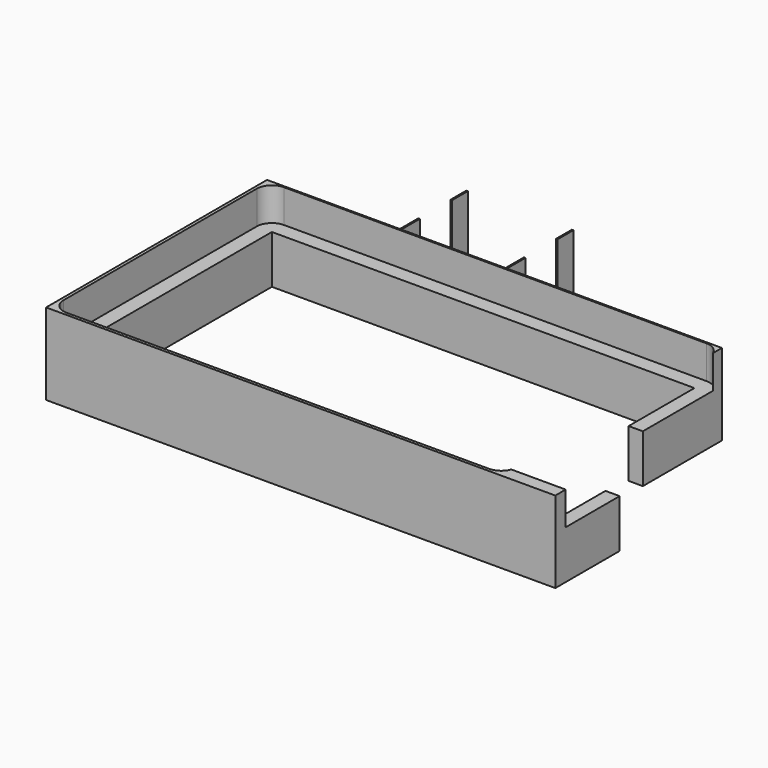
from build123d import *

# Parameters (mm, degrees)
F0_W          = 170
F0_H          = 130
F1_DEPTH      = 34
F2_T          = -1
F3_W          = 43.5
F3_H          = 38
F4_DEPTH      = 32
F5_T          = 0.5
F5_T3_DEPTH   = 34
F5_T5_DEPTH   = 125.5
F5_T7_DEPTH   = 33
F5_T9_DEPTH   = 2
F5_T11_DEPTH  = 129
F5_T13_DEPTH  = 169
F5_T15_DEPTH  = 91
F5_T17_DEPTH  = 44.5
F5_T19_DEPTH  = 39
F6_W          = 35
F6_H          = 38
F7_DEPTH      = 32
F8_T          = 0.5
F8_T3_DEPTH   = 2
F8_T5_DEPTH   = 33
F8_T7_DEPTH   = 91
F8_T9_DEPTH   = 34
F8_T11_DEPTH  = 79.5
F8_T13_DEPTH  = 169
F8_T15_DEPTH  = 129
F8_T17_DEPTH  = 90.5
F8_T19_DEPTH  = 39
F8_T21_DEPTH  = 44.5
F8_T23_DEPTH  = 33.5
F8_T25_DEPTH  = 1.5
F8_T27_DEPTH  = 39
F8_T29_DEPTH  = 33
F8_T31_DEPTH  = 1.5
F8_T33_DEPTH  = 1.5
F8_T35_DEPTH  = 38.5
F8_T37_DEPTH  = 1.5000245068
F8_T39_DEPTH  = 1.5000245068
F8_T41_DEPTH  = 44
F9_W          = 89.5
F9_H          = 38
F10_DEPTH     = 32
F11_T         = 0.5
F11_T3_DEPTH  = 2
F11_T5_DEPTH  = 33
F11_T7_DEPTH  = 91
F11_T9_DEPTH  = 34
F11_T11_DEPTH = 169
F11_T13_DEPTH = 44.5
F11_T15_DEPTH = 33.5
F11_T17_DEPTH = 1.5
F11_T19_DEPTH = 39
F11_T21_DEPTH = 33
F11_T23_DEPTH = 1.5
F11_T25_DEPTH = 1.5
F11_T27_DEPTH = 38.5
F11_T29_DEPTH = 1.5000245068
F11_T31_DEPTH = 1.5000245068
F11_T33_DEPTH = 44
F11_T35_DEPTH = 35.5
F12_W         = 150
F12_H         = 90
F13_DEPTH     = 32
F15_DEPTH     = 17
F16_W         = 140
F16_H         = 80
F17_DEPTH     = 25
F18_DEPTH     = 25
F19_DEPTH     = 25
F20_DEPTH     = 25
F21_DEPTH     = 25
F24_W         = 170
F24_H         = 34
F25_DEPTH     = 11
F26_W         = 119
F26_H         = 34
F27_DEPTH     = 19.3
F28_W         = 32.0991082117
F28_H         = 16
F29_DEPTH     = 25
F30_W         = 13.2916904986
F30_H         = 28.4444186985
F31_DEPTH     = 96.3
F32_W         = 236.7293909192
F32_H         = 199.1855278611
F33_DEPTH     = 7
F34_DEPTH     = 18
F35_DEPTH     = 18
F36_DEPTH     = 27.5


# Not quite as in the source:
# - a feature of the source that left no trace in its solid (it failed there, or was rolled back) is left out
# - a shell that OpenCascade refuses in one call is made with other operations: the cavity is built on its own and cut out


with BuildPart() as f1:
    # F0 (on Top) → F1 (new body)
    with BuildSketch(Plane.XY):
        with Locations((-10.1464114764, -3.7471540272)):
            Rectangle(F0_W, F0_H)
    extrude(amount=F1_DEPTH)

    # F2
    f2_openings = [f1.faces().sort_by_distance(p)[0] for p in [
        (-10.146411, -3.747154, 34),
    ]]
    offset(amount=F2_T, openings=f2_openings)

    # F3 (on face) → F4 (join)
    with BuildSketch(Plane.XY.offset(1)):
        with Locations((-72.3964114764, 41.2528459728)):
            Rectangle(F3_W, F3_H)
    extrude(amount=F4_DEPTH)

    # F5: shell of thickness 0.5, made by hand


with BuildPart() as f5_core1:
    # F5_t2: copy of F1
    add(f1.part)

    # the walls: a layer under each face that stays
    f5_faces = [f5_core1.faces().sort_by_distance(p)[0] for p in [
        (-10.1464114764, 61.2528459728, 17),
        (74.8535885236, -3.7471540272, 17),
        (-95.1464114764, -3.7471540272, 17),
        (-10.1464114764, -3.7471540272, 0),
        (-3.5057864764, -68.2121746034, 34),
        (-10.1464114764, -68.7471540272, 17),
        (-10.1464114764, 60.2528459728, 17.5),
        (73.8535885236, -3.7471540272, 17.5),
        (-10.1464114764, -67.7471540272, 17.5),
        (-94.1464114764, -3.7471540272, 17.5),
        (-10.1464114764, -3.7471540272, 1),
        (-50.6464114764, 41.2528459728, 17),
        (-72.3964114764, 22.2528459728, 17),
    ]]
    thicken(f5_faces, amount=-F5_T, mode=Mode.SUBTRACT)

    # F5_s4 → F5_t3 (cut)
    with BuildSketch(Plane.XY.offset(0.5)):
        Polygon((73.8485885236, 60.2478459728), (73.8535885236, 60.7528459728), (74.3535885236, 60.7528459728), (74.3535885236, 60.2528459728), align=None)
        Polygon((73.8485885236, -67.7421540272), (74.3535885236, -67.7471540272), (74.3535885236, -68.2471540272), (73.8535885236, -68.2471540272), align=None)
        Polygon((-94.1414114764, -67.7421540272), (-94.1464114764, -68.2471540272), (-94.6464114764, -68.2471540272), (-94.6464114764, -67.7471540272), align=None)
    extrude(amount=F5_T3_DEPTH, mode=Mode.SUBTRACT)

    # F5_s6 → F5_t5 (cut)
    with BuildSketch(Plane.YZ.offset(-51.1464114764)):
        Polygon((60.2478459728, 1.005), (60.7528459728, 1), (60.7528459728, 0.5), (60.2528459728, 0.5), align=None)
    extrude(amount=F5_T5_DEPTH, mode=Mode.SUBTRACT)

    # F5_s8 → F5_t7 (cut)
    with BuildSketch(Plane.XY.offset(0.5)):
        Polygon((-50.6414114764, 60.2478459728), (-50.6464114764, 60.7528459728), (-51.1464114764, 60.7528459728), (-51.1464114764, 60.2528459728), align=None)
        Polygon((-94.1414114764, 22.2478459728), (-94.6464114764, 22.2528459728), (-94.6464114764, 22.7528459728), (-94.1464114764, 22.7528459728), align=None)
    extrude(amount=F5_T7_DEPTH, mode=Mode.SUBTRACT)

    # F5_s10 → F5_t9 (cut)
    with BuildSketch(Plane.XY.offset(32.5)):
        Polygon((-94.1414114764, 60.2478459728), (-94.1464114764, 60.7528459728), (-94.6464114764, 60.7528459728), (-94.6464114764, 60.2528459728), align=None)
    extrude(amount=F5_T9_DEPTH, mode=Mode.SUBTRACT)

    # F5_s12 → F5_t11 (cut)
    with BuildSketch(Plane.XZ.offset(-60.7528459728)):
        Polygon((73.8485885236, 1.005), (74.3535885236, 1), (74.3535885236, 0.5), (73.8535885236, 0.5), align=None)
    extrude(amount=F5_T11_DEPTH, mode=Mode.SUBTRACT)

    # F5_s14 → F5_t13 (cut)
    with BuildSketch(Plane.YZ.offset(-94.6464114764)):
        Polygon((-67.7421540272, 1.005), (-68.2471540272, 1), (-68.2471540272, 0.5), (-67.7471540272, 0.5), align=None)
    extrude(amount=F5_T13_DEPTH, mode=Mode.SUBTRACT)

    # F5_s16 → F5_t15 (cut)
    with BuildSketch(Plane.XZ.offset(-22.7528459728)):
        Polygon((-94.1414114764, 1.005), (-94.6464114764, 1), (-94.6464114764, 0.5), (-94.1464114764, 0.5), align=None)
    extrude(amount=F5_T15_DEPTH, mode=Mode.SUBTRACT)

    # F5_s18 → F5_t17 (cut)
    with BuildSketch(Plane.YZ.offset(-94.6464114764)):
        Polygon((22.2478459728, 1.005), (22.2528459728, 0.5), (22.7528459728, 0.5), (22.7528459728, 1), align=None)
    extrude(amount=F5_T17_DEPTH, mode=Mode.SUBTRACT)

    # F5_s20 → F5_t19 (cut)
    with BuildSketch(Plane.XZ.offset(-60.7528459728)):
        Polygon((-50.6414114764, 1.005), (-50.6464114764, 0.5), (-51.1464114764, 0.5), (-51.1464114764, 1), align=None)
    extrude(amount=F5_T19_DEPTH, mode=Mode.SUBTRACT)


with BuildPart() as f1_1:
    add(f1.part)

    # what is left inside the walls is the cavity
    f5_cavity = [f5_core1.part.solids().sort_by_distance(p)[0] for p in [
        (-72.896411, 35.419513, 0.505),
    ]]
    add(f5_cavity, mode=Mode.SUBTRACT)

    # F6 (on face) → F7 (join)
    with BuildSketch(Plane.XY.offset(1)):
        with Locations((-33.1464114764, 41.2528459728)):
            Rectangle(F6_W, F6_H)
    extrude(amount=F7_DEPTH)

    # F8: shell of thickness 0.5, made by hand


with BuildPart() as f8_core1:
    # F8_t2: copy of F1
    add(f1_1.part)

    # the walls: a layer under each face that stays
    f8_faces = [f8_core1.faces().sort_by_distance(p)[0] for p in [
        (-10.1464114764, 61.2528459728, 17),
        (-3.5057864764, -68.2121746034, 34),
        (-94.1464114764, -3.7471540272, 17.5),
        (-10.1464114764, -3.7471540272, 1),
        (-15.6464114764, 41.2528459728, 17),
        (-54.8964114764, 22.2528459728, 17),
        (-72.8964114764, 22.7528459728, 16.75),
        (-94.6464114764, 41.7528459728, 16.75),
        (-94.3939114764, 60.2503459728, 32.75),
        (-94.1439114764, 60.5003459728, 32.75),
        (-72.6464114764, 60.5028459728, 33),
        (-94.3939114764, 60.5003459728, 32.5),
        (-72.8964114764, 60.7528459728, 16.75),
        (-72.8964114764, 41.7528459728, 0.5),
        (-51.1464114764, 41.7528459728, 16.75),
        (-94.3964114764, 41.5028459728, 33),
        (-10.1464114764, -67.7471540272, 17.5),
        (73.8535885236, -3.7471540272, 17.5),
        (-10.1464114764, 60.2528459728, 17.5),
        (-10.1464114764, -68.7471540272, 17),
        (-10.1464114764, -3.7471540272, 0),
        (-95.1464114764, -3.7471540272, 17),
        (74.8535885236, -3.7471540272, 17),
    ]]
    thicken(f8_faces, amount=-F8_T, mode=Mode.SUBTRACT)

    # F8_s4 → F8_t3 (cut)
    with BuildSketch(Plane.XY.offset(32.5)):
        Polygon((-94.1414114764, 60.2478459728), (-94.6464114764, 60.2528459728), (-94.6464114764, 60.7528459728), (-94.1464114764, 60.7528459728), align=None)
    extrude(amount=F8_T3_DEPTH, mode=Mode.SUBTRACT)

    # F8_s6 → F8_t5 (cut)
    with BuildSketch(Plane.XY.offset(0.5)):
        Polygon((-94.1414114764, 22.2478459728), (-94.6464114764, 22.2528459728), (-94.6464114764, 22.7528459728), (-94.1464114764, 22.7528459728), align=None)
        Polygon((-15.6414114764, 60.2478459728), (-16.1464114764, 60.2528459728), (-16.1464114764, 60.7528459728), (-15.6464114764, 60.7528459728), align=None)
    extrude(amount=F8_T5_DEPTH, mode=Mode.SUBTRACT)

    # F8_s8 → F8_t7 (cut)
    with BuildSketch(Plane.XZ.offset(-22.7528459728)):
        Polygon((-94.1414114764, 1.005), (-94.6464114764, 1), (-94.6464114764, 0.5), (-94.1464114764, 0.5), align=None)
    extrude(amount=F8_T7_DEPTH, mode=Mode.SUBTRACT)

    # F8_s10 → F8_t9 (cut)
    with BuildSketch(Plane.XY.offset(0.5)):
        Polygon((-94.1414114764, -67.7421540272), (-94.6464114764, -67.7471540272), (-94.6464114764, -68.2471540272), (-94.1464114764, -68.2471540272), align=None)
        Polygon((73.8485885236, -67.7421540272), (73.8535885236, -68.2471540272), (74.3535885236, -68.2471540272), (74.3535885236, -67.7471540272), align=None)
        Polygon((73.8485885236, 60.2478459728), (74.3535885236, 60.2528459728), (74.3535885236, 60.7528459728), (73.8535885236, 60.7528459728), align=None)
    extrude(amount=F8_T9_DEPTH, mode=Mode.SUBTRACT)

    # F8_s12 → F8_t11 (cut)
    with BuildSketch(Plane.YZ.offset(-94.6464114764)):
        Polygon((22.2478459728, 1.005), (22.2528459728, 0.5), (22.7528459728, 0.5), (22.7528459728, 1), align=None)
    extrude(amount=F8_T11_DEPTH, mode=Mode.SUBTRACT)

    # F8_s14 → F8_t13 (cut)
    with BuildSketch(Plane.YZ.offset(-94.6464114764)):
        Polygon((-67.7421540272, 1.005), (-67.7471540272, 0.5), (-68.2471540272, 0.5), (-68.2471540272, 1), align=None)
    extrude(amount=F8_T13_DEPTH, mode=Mode.SUBTRACT)

    # F8_s16 → F8_t15 (cut)
    with BuildSketch(Plane.XZ.offset(-60.7528459728)):
        Polygon((73.8485885236, 1.005), (73.8535885236, 0.5), (74.3535885236, 0.5), (74.3535885236, 1), align=None)
    extrude(amount=F8_T15_DEPTH, mode=Mode.SUBTRACT)

    # F8_s18 → F8_t17 (cut)
    with BuildSketch(Plane.YZ.offset(-16.1464114764)):
        Polygon((60.2478459728, 1.005), (60.2528459728, 0.5), (60.7528459728, 0.5), (60.7528459728, 1), align=None)
    extrude(amount=F8_T17_DEPTH, mode=Mode.SUBTRACT)

    # F8_s20 → F8_t19 (cut)
    with BuildSketch(Plane.XZ.offset(-60.7528459728)):
        Polygon((-15.6414114764, 1.005), (-15.6464114764, 0.5), (-16.1464114764, 0.5), (-16.1464114764, 1), align=None)
    extrude(amount=F8_T19_DEPTH, mode=Mode.SUBTRACT)

    # F8_s22 → F8_t21 (cut)
    with BuildSketch(Plane.YZ.offset(-95.1464114764)):
        Polygon((22.7578459728, 0.505), (22.2528459728, 0.5), (22.2528459728, 0), (22.7528459728, 0), align=None)
        Polygon((60.7478459728, 0.505), (61.2528459728, 0.5), (61.2528459728, 0), (60.7528459728, 0), align=None)
    extrude(amount=F8_T21_DEPTH, mode=Mode.SUBTRACT)

    # F8_s24 → F8_t23 (cut)
    with BuildSketch(Plane.XY):
        Polygon((-94.6414114764, 22.7578459728), (-94.6464114764, 22.2528459728), (-95.1464114764, 22.2528459728), (-95.1464114764, 22.7528459728), align=None)
        Polygon((-51.1514114764, 22.7578459728), (-51.1464114764, 22.2528459728), (-50.6464114764, 22.2528459728), (-50.6464114764, 22.7528459728), align=None)
        Polygon((-51.1514114764, 60.7478459728), (-51.1464114764, 61.2528459728), (-50.6464114764, 61.2528459728), (-50.6464114764, 60.7528459728), align=None)
    extrude(amount=F8_T23_DEPTH, mode=Mode.SUBTRACT)

    # F8_s26 → F8_t25 (cut)
    with BuildSketch(Plane.YZ.offset(-95.1464114764)):
        Polygon((22.7578459728, 32.995), (22.2528459728, 33), (22.2528459728, 33.5), (22.7528459728, 33.5), align=None)
        Polygon((60.7478459728, 32.495), (60.7528459728, 33), (61.2528459728, 33), (61.2528459728, 32.5), align=None)
    extrude(amount=F8_T25_DEPTH, mode=Mode.SUBTRACT)

    # F8_s28 → F8_t27 (cut)
    with BuildSketch(Plane.XZ.offset(-61.2528459728)):
        Polygon((-94.6414114764, 0.505), (-95.1464114764, 0.5), (-95.1464114764, 0), (-94.6464114764, 0), align=None)
        Polygon((-51.1514114764, 0.505), (-51.1464114764, 0), (-50.6464114764, 0), (-50.6464114764, 0.5), align=None)
    extrude(amount=F8_T27_DEPTH, mode=Mode.SUBTRACT)

    # F8_s30 → F8_t29 (cut)
    with BuildSketch(Plane.XY):
        Polygon((-94.6414114764, 60.7478459728), (-95.1464114764, 60.7528459728), (-95.1464114764, 61.2528459728), (-94.6464114764, 61.2528459728), align=None)
    extrude(amount=F8_T29_DEPTH, mode=Mode.SUBTRACT)

    # F8_s32 → F8_t31 (cut)
    with BuildSketch(Plane.XZ.offset(-61.2528459728)):
        Polygon((-94.6414114764, 32.495), (-95.1464114764, 32.5), (-95.1464114764, 33), (-94.6464114764, 33), align=None)
        Polygon((-51.1514114764, 32.995), (-51.1464114764, 33.5), (-50.6464114764, 33.5), (-50.6464114764, 33), align=None)
    extrude(amount=F8_T31_DEPTH, mode=Mode.SUBTRACT)

    # F8_s34 → F8_t33 (cut)
    with BuildSketch(Plane.XY.offset(32)):
        Polygon((-94.6414609789, 60.2478462179), (-95.1464114764, 60.2528459728), (-95.1464114764, 60.7578209747), (-94.641461224, 60.7528214672), align=None)
        Polygon((-94.1414117215, 60.7478954753), (-94.6463869708, 60.7478957204), (-94.6513864783, 61.2528459728), (-94.1464114764, 61.2528459728), align=None)
    extrude(amount=F8_T33_DEPTH, mode=Mode.SUBTRACT)

    # F8_s36 → F8_t35 (cut)
    with BuildSketch(Plane.XZ.offset(-60.7528459728)):
        Polygon((-94.6414114764, 32.995), (-95.1464114764, 33), (-95.1464114764, 33.5), (-94.6464114764, 33.5), align=None)
    extrude(amount=F8_T35_DEPTH, mode=Mode.SUBTRACT)

    # F8_s38 → F8_t37 (cut)
    with BuildSketch(Plane(origin=(-95.7336140862, 0.9478575652, 0), x_dir=(0, 0, 1), z_dir=(0.9999509888, -0.0099005048, 0))):
        Polygon((32.995, -59.3078456537), (33, -59.8128456537), (33.5, -59.8128456537), (33.5, -59.3128456537), align=None)
    extrude(amount=F8_T37_DEPTH, mode=Mode.SUBTRACT)

    # F8_s40 → F8_t39 (cut)
    with BuildSketch(Plane(origin=(-0.6007818495, 60.6789668039, 0), x_dir=(0, 0, 1), z_dir=(-0.0099005048, 0.9999509888, 0))):
        Polygon((32.995, -93.5353134023), (33, -94.0403134023), (33.5, -94.0403134023), (33.5, -93.5403134023), align=None)
    extrude(amount=F8_T39_DEPTH, mode=Mode.SUBTRACT)

    # F8_s42 → F8_t41 (cut)
    with BuildSketch(Plane.YZ.offset(-94.6464114764)):
        Polygon((60.7478459728, 32.995), (60.7528459728, 33.5), (61.2528459728, 33.5), (61.2528459728, 33), align=None)
    extrude(amount=F8_T41_DEPTH, mode=Mode.SUBTRACT)


with BuildPart() as f1_2:
    add(f1_1.part)

    # what is left inside the walls is the cavity
    f8_cavity = [f8_core1.part.solids().sort_by_distance(p)[0] for p in [
        (-33.396411, 35.419513, 32.995),
    ]]
    add(f8_cavity, mode=Mode.SUBTRACT)

    # F9 (on face) → F10 (join)
    with BuildSketch(Plane.XY.offset(1)):
        with Locations((29.1035885236, 41.2528459728)):
            Rectangle(F9_W, F9_H)
    extrude(amount=F10_DEPTH)

    # F11: shell of thickness 0.5, made by hand


with BuildPart() as f11_core1:
    # F11_t2: copy of F1
    add(f1_2.part)

    # the walls: a layer under each face that stays
    f11_faces = [f11_core1.faces().sort_by_distance(p)[0] for p in [
        (-10.1464114764, 61.2528459728, 17),
        (-3.5057864764, -68.2121746034, 34),
        (-94.1464114764, -3.7471540272, 17.5),
        (-10.1464114764, -22.7471540272, 1),
        (-10.1464114764, 22.2528459728, 17),
        (-72.8964114764, 22.7528459728, 16.75),
        (-94.6464114764, 41.7528459728, 16.75),
        (-94.3939114764, 60.2503459728, 32.75),
        (-94.1439114764, 60.5003459728, 32.75),
        (-72.6464114764, 60.5028459728, 33),
        (-94.3939114764, 60.5003459728, 32.5),
        (-72.8964114764, 60.7528459728, 16.75),
        (-72.8964114764, 41.7528459728, 0.5),
        (-51.1464114764, 41.7528459728, 16.75),
        (-50.6464114764, 41.7528459728, 16.75),
        (-33.3964114764, 60.7528459728, 16.75),
        (-33.3964114764, 41.7528459728, 0.5),
        (-33.3964114764, 60.5028459728, 33),
        (-33.3964114764, 22.7528459728, 16.75),
        (-16.1464114764, 41.7528459728, 16.75),
        (-94.3964114764, 41.5028459728, 33),
        (-10.1464114764, -67.7471540272, 17.5),
        (73.8535885236, -3.7471540272, 17.5),
        (-10.1464114764, 60.2528459728, 33.5),
        (-10.1464114764, -68.7471540272, 17),
        (-10.1464114764, -3.7471540272, 0),
        (-95.1464114764, -3.7471540272, 17),
        (74.8535885236, -3.7471540272, 17),
    ]]
    thicken(f11_faces, amount=-F11_T, mode=Mode.SUBTRACT)

    # F11_s4 → F11_t3 (cut)
    with BuildSketch(Plane.XY.offset(32.5)):
        Polygon((-94.1414114764, 60.2478459728), (-94.6464114764, 60.2528459728), (-94.6464114764, 60.7528459728), (-94.1464114764, 60.7528459728), align=None)
        Polygon((73.8485885236, 60.2478459728), (74.3535885236, 60.2528459728), (74.3535885236, 60.7528459728), (73.8535885236, 60.7528459728), align=None)
    extrude(amount=F11_T3_DEPTH, mode=Mode.SUBTRACT)

    # F11_s6 → F11_t5 (cut)
    with BuildSketch(Plane.XY.offset(0.5)):
        Polygon((-94.1414114764, 22.2478459728), (-94.6464114764, 22.2528459728), (-94.6464114764, 22.7528459728), (-94.1464114764, 22.7528459728), align=None)
        Polygon((73.8485885236, 22.2478459728), (73.8535885236, 22.7528459728), (74.3535885236, 22.7528459728), (74.3535885236, 22.2528459728), align=None)
    extrude(amount=F11_T5_DEPTH, mode=Mode.SUBTRACT)

    # F11_s8 → F11_t7 (cut)
    with BuildSketch(Plane.XZ.offset(-22.7528459728)):
        Polygon((-94.1414114764, 1.005), (-94.6464114764, 1), (-94.6464114764, 0.5), (-94.1464114764, 0.5), align=None)
        Polygon((73.8485885236, 1.005), (73.8535885236, 0.5), (74.3535885236, 0.5), (74.3535885236, 1), align=None)
    extrude(amount=F11_T7_DEPTH, mode=Mode.SUBTRACT)

    # F11_s10 → F11_t9 (cut)
    with BuildSketch(Plane.XY.offset(0.5)):
        Polygon((-94.1414114764, -67.7421540272), (-94.6464114764, -67.7471540272), (-94.6464114764, -68.2471540272), (-94.1464114764, -68.2471540272), align=None)
        Polygon((73.8485885236, -67.7421540272), (73.8535885236, -68.2471540272), (74.3535885236, -68.2471540272), (74.3535885236, -67.7471540272), align=None)
    extrude(amount=F11_T9_DEPTH, mode=Mode.SUBTRACT)

    # F11_s12 → F11_t11 (cut)
    with BuildSketch(Plane.YZ.offset(-94.6464114764)):
        Polygon((22.2478459728, 1.005), (22.2528459728, 0.5), (22.7528459728, 0.5), (22.7528459728, 1), align=None)
        Polygon((-67.7421540272, 1.005), (-67.7471540272, 0.5), (-68.2471540272, 0.5), (-68.2471540272, 1), align=None)
    extrude(amount=F11_T11_DEPTH, mode=Mode.SUBTRACT)

    # F11_s14 → F11_t13 (cut)
    with BuildSketch(Plane.YZ.offset(-95.1464114764)):
        Polygon((22.7578459728, 0.505), (22.2528459728, 0.5), (22.2528459728, 0), (22.7528459728, 0), align=None)
        Polygon((60.7478459728, 0.505), (61.2528459728, 0.5), (61.2528459728, 0), (60.7528459728, 0), align=None)
    extrude(amount=F11_T13_DEPTH, mode=Mode.SUBTRACT)

    # F11_s16 → F11_t15 (cut)
    with BuildSketch(Plane.XY):
        Polygon((-94.6414114764, 22.7578459728), (-94.6464114764, 22.2528459728), (-95.1464114764, 22.2528459728), (-95.1464114764, 22.7528459728), align=None)
        Polygon((-51.1514114764, 22.7578459728), (-51.1464114764, 22.2528459728), (-50.6464114764, 22.2528459728), (-50.6464114764, 22.7528459728), align=None)
        Polygon((-51.1514114764, 60.7478459728), (-51.1464114764, 61.2528459728), (-50.6464114764, 61.2528459728), (-50.6464114764, 60.7528459728), align=None)
        Polygon((-50.6414114764, 22.7578459728), (-51.1464114764, 22.7528459728), (-51.1464114764, 22.2528459728), (-50.6464114764, 22.2528459728), align=None)
        Polygon((-50.6414114764, 60.7478459728), (-51.1464114764, 60.7528459728), (-51.1464114764, 61.2528459728), (-50.6464114764, 61.2528459728), align=None)
        Polygon((-16.1514114764, 60.7478459728), (-16.1464114764, 61.2528459728), (-15.6464114764, 61.2528459728), (-15.6464114764, 60.7528459728), align=None)
        Polygon((-16.1514114764, 22.7578459728), (-16.1464114764, 22.2528459728), (-15.6464114764, 22.2528459728), (-15.6464114764, 22.7528459728), align=None)
    extrude(amount=F11_T15_DEPTH, mode=Mode.SUBTRACT)

    # F11_s18 → F11_t17 (cut)
    with BuildSketch(Plane.YZ.offset(-95.1464114764)):
        Polygon((22.7578459728, 32.995), (22.2528459728, 33), (22.2528459728, 33.5), (22.7528459728, 33.5), align=None)
        Polygon((60.7478459728, 32.495), (60.7528459728, 33), (61.2528459728, 33), (61.2528459728, 32.5), align=None)
    extrude(amount=F11_T17_DEPTH, mode=Mode.SUBTRACT)

    # F11_s20 → F11_t19 (cut)
    with BuildSketch(Plane.XZ.offset(-61.2528459728)):
        Polygon((-94.6414114764, 0.505), (-95.1464114764, 0.5), (-95.1464114764, 0), (-94.6464114764, 0), align=None)
        Polygon((-51.1514114764, 0.505), (-51.1464114764, 0), (-50.6464114764, 0), (-50.6464114764, 0.5), align=None)
        Polygon((-50.6414114764, 0.505), (-51.1464114764, 0.5), (-51.1464114764, 0), (-50.6464114764, 0), align=None)
        Polygon((-16.1514114764, 0.505), (-16.1464114764, 0), (-15.6464114764, 0), (-15.6464114764, 0.5), align=None)
    extrude(amount=F11_T19_DEPTH, mode=Mode.SUBTRACT)

    # F11_s22 → F11_t21 (cut)
    with BuildSketch(Plane.XY):
        Polygon((-94.6414114764, 60.7478459728), (-95.1464114764, 60.7528459728), (-95.1464114764, 61.2528459728), (-94.6464114764, 61.2528459728), align=None)
    extrude(amount=F11_T21_DEPTH, mode=Mode.SUBTRACT)

    # F11_s24 → F11_t23 (cut)
    with BuildSketch(Plane.XZ.offset(-61.2528459728)):
        Polygon((-94.6414114764, 32.495), (-95.1464114764, 32.5), (-95.1464114764, 33), (-94.6464114764, 33), align=None)
        Polygon((-51.1514114764, 32.995), (-51.1464114764, 33.5), (-50.6464114764, 33.5), (-50.6464114764, 33), align=None)
        Polygon((-50.6414114764, 32.995), (-51.1464114764, 33), (-51.1464114764, 33.5), (-50.6464114764, 33.5), align=None)
        Polygon((-16.1514114764, 32.995), (-16.1464114764, 33.5), (-15.6464114764, 33.5), (-15.6464114764, 33), align=None)
    extrude(amount=F11_T23_DEPTH, mode=Mode.SUBTRACT)

    # F11_s26 → F11_t25 (cut)
    with BuildSketch(Plane.XY.offset(32)):
        Polygon((-94.6414609789, 60.2478462179), (-95.1464114764, 60.2528459728), (-95.1464114764, 60.7578209747), (-94.641461224, 60.7528214672), align=None)
        Polygon((-94.1414117215, 60.7478954753), (-94.6463869708, 60.7478957204), (-94.6513864783, 61.2528459728), (-94.1464114764, 61.2528459728), align=None)
    extrude(amount=F11_T25_DEPTH, mode=Mode.SUBTRACT)

    # F11_s28 → F11_t27 (cut)
    with BuildSketch(Plane.XZ.offset(-60.7528459728)):
        Polygon((-94.6414114764, 32.995), (-95.1464114764, 33), (-95.1464114764, 33.5), (-94.6464114764, 33.5), align=None)
    extrude(amount=F11_T27_DEPTH, mode=Mode.SUBTRACT)

    # F11_s30 → F11_t29 (cut)
    with BuildSketch(Plane(origin=(-95.7336140862, 0.9478575652, 0), x_dir=(0, 0, 1), z_dir=(0.9999509888, -0.0099005048, 0))):
        Polygon((32.995, -59.3078456537), (33, -59.8128456537), (33.5, -59.8128456537), (33.5, -59.3128456537), align=None)
    extrude(amount=F11_T29_DEPTH, mode=Mode.SUBTRACT)

    # F11_s32 → F11_t31 (cut)
    with BuildSketch(Plane(origin=(-0.6007818495, 60.6789668039, 0), x_dir=(0, 0, 1), z_dir=(-0.0099005048, 0.9999509888, 0))):
        Polygon((32.995, -93.5353134023), (33, -94.0403134023), (33.5, -94.0403134023), (33.5, -93.5403134023), align=None)
    extrude(amount=F11_T31_DEPTH, mode=Mode.SUBTRACT)

    # F11_s34 → F11_t33 (cut)
    with BuildSketch(Plane.YZ.offset(-94.6464114764)):
        Polygon((60.7478459728, 32.995), (60.7528459728, 33.5), (61.2528459728, 33.5), (61.2528459728, 33), align=None)
    extrude(amount=F11_T33_DEPTH, mode=Mode.SUBTRACT)

    # F11_s36 → F11_t35 (cut)
    with BuildSketch(Plane.YZ.offset(-51.1464114764)):
        Polygon((60.7478459728, 0.505), (61.2528459728, 0.5), (61.2528459728, 0), (60.7528459728, 0), align=None)
        Polygon((60.7478459728, 32.995), (61.2528459728, 33), (61.2528459728, 33.5), (60.7528459728, 33.5), align=None)
        Polygon((22.7578459728, 0.505), (22.7528459728, 0), (22.2528459728, 0), (22.2528459728, 0.5), align=None)
    extrude(amount=F11_T35_DEPTH, mode=Mode.SUBTRACT)


with BuildPart() as f1_3:
    add(f1_2.part)

    # what is left inside the walls is the cavity
    f11_cavity = [f11_core1.part.solids().sort_by_distance(p)[0] for p in [
        (29.353589, 35.419513, 0.505),
    ]]
    add(f11_cavity, mode=Mode.SUBTRACT)

    # F12 (on face) → F13 (join)
    with BuildSketch(Plane.XY.offset(1)):
        with Locations((-19.1464114764, -22.7471540272)):
            Rectangle(F12_W, F12_H)
    extrude(amount=F13_DEPTH)

    # F14 (on face) → F15 (cut)
    with BuildSketch(Plane.XY.offset(33)):
        with BuildLine():
            Line((50.8535885236, 22.2528459728), (-89.1464114764, 22.2528459728))
            ThreePointArc((-89.1464114764, 22.2528459728), (-92.6819453823, 20.7883798787), (-94.1464114764, 17.2528459728))
            Line((-94.1464114764, 17.2528459728), (-94.1464114764, -62.7471540272))
            ThreePointArc((-94.1464114764, -62.7471540272), (-92.6819453823, -66.2826879332), (-89.1464114764, -67.7471540272))
            Line((-89.1464114764, -67.7471540272), (50.8535885236, -67.7471540272))
            ThreePointArc((50.8535885236, -67.7471540272), (54.3891224295, -66.2826879332), (55.8535885236, -62.7471540272))
            Line((55.8535885236, -62.7471540272), (55.8535885236, 17.2528459728))
            ThreePointArc((55.8535885236, 17.2528459728), (54.3891224295, 20.7883798787), (50.8535885236, 22.2528459728))
        make_face()
    extrude(amount=-F15_DEPTH, mode=Mode.SUBTRACT)

    # F16 (on face) → F17 (cut)
    with BuildSketch(Plane.XY.offset(16)):
        with Locations((-19.1464114764, -22.7471540272)):
            Rectangle(F16_W, F16_H)
    extrude(amount=-F17_DEPTH, mode=Mode.SUBTRACT)

    # F18 (cut): a face of the model
    f18_faces = [f1_3.faces().sort_by_distance(p)[0] for p in [
        (-72.8964114764, 41.7528459728, 0.5),
    ]]
    extrude(f18_faces, amount=-F18_DEPTH, mode=Mode.SUBTRACT)

    # F19 (cut): a face of the model
    f19_faces = [f1_3.faces().sort_by_distance(p)[0] for p in [
        (-33.3964114764, 41.7528459728, 0.5),
    ]]
    extrude(f19_faces, amount=-F19_DEPTH, mode=Mode.SUBTRACT)

    # F20 (cut): a face of the model
    f20_faces = [f1_3.faces().sort_by_distance(p)[0] for p in [
        (29.3535885236, 41.7528459728, 0.5),
    ]]
    extrude(f20_faces, amount=-F20_DEPTH, mode=Mode.SUBTRACT)

    # F21 (cut): a face of the model
    f21_faces = [f1_3.faces().sort_by_distance(p)[0] for p in [
        (64.8535885236, -22.7471540272, 1),
    ]]
    extrude(f21_faces, amount=-F21_DEPTH, mode=Mode.SUBTRACT)

    # F24 (on face) → F25 (cut)
    with BuildSketch(Plane(origin=(0, 61.2528459728, 0), x_dir=(-1, 0, 0), z_dir=(0, 1, 0))):
        with Locations((10.1464114764, 17)):
            Rectangle(F24_W, F24_H)
    extrude(amount=-F25_DEPTH, mode=Mode.SUBTRACT)

    # F26 (on face) → F27 (cut)
    with BuildSketch(Plane.YZ.offset(74.8535885236)):
        with Locations((-9.2471540272, 17)):
            Rectangle(F26_W, F26_H)
    extrude(amount=-F27_DEPTH, mode=Mode.SUBTRACT)

    # F28 (on face) → F29 (cut)
    with BuildSketch(Plane.YZ.offset(55.5535885236)):
        with Locations((-26.0480144061, 8)):
            Rectangle(F28_W, F28_H)
    extrude(amount=-F29_DEPTH, mode=Mode.SUBTRACT)

    # F30 (on face) → F31 (cut)
    with BuildSketch(Plane(origin=(-95.1464114764, 0, 0), x_dir=(0, -1, 0), z_dir=(-1, 0, 0))):
        with Locations((-37.051377818, 19.7777906507)):
            Rectangle(F30_W, F30_H)
    extrude(amount=-F31_DEPTH, mode=Mode.SUBTRACT)

    # F32 (on face) → F33 (cut)
    with BuildSketch(Plane.XY.offset(34)):
        with Locations((13.9653496444, 0.8634440601)):
            Rectangle(F32_W, F32_H)
    extrude(amount=-F33_DEPTH, mode=Mode.SUBTRACT)

    # F34 (add): a face of the model
    f34_faces = [f1_3.faces().sort_by_distance(p)[0] for p in [
        (55.5535885236, -56.5371257993, 9.346366631),
    ]]
    extrude(f34_faces, amount=F34_DEPTH)

    # F35 (cut): a face of the model
    f35_faces = [f1_3.faces().sort_by_distance(p)[0] for p in [
        (50.8535885236, -52.4223612696, 8),
    ]]
    extrude(f35_faces, amount=-F35_DEPTH, mode=Mode.SUBTRACT)

    # F36 (cut): a face of the model
    f36_faces = [f1_3.faces().sort_by_distance(p)[0] for p in [
        (-94.8964114764, 50.2528459728, 13.5),
    ]]
    extrude(f36_faces, amount=-F36_DEPTH, mode=Mode.SUBTRACT)


solid = f1_3.part
